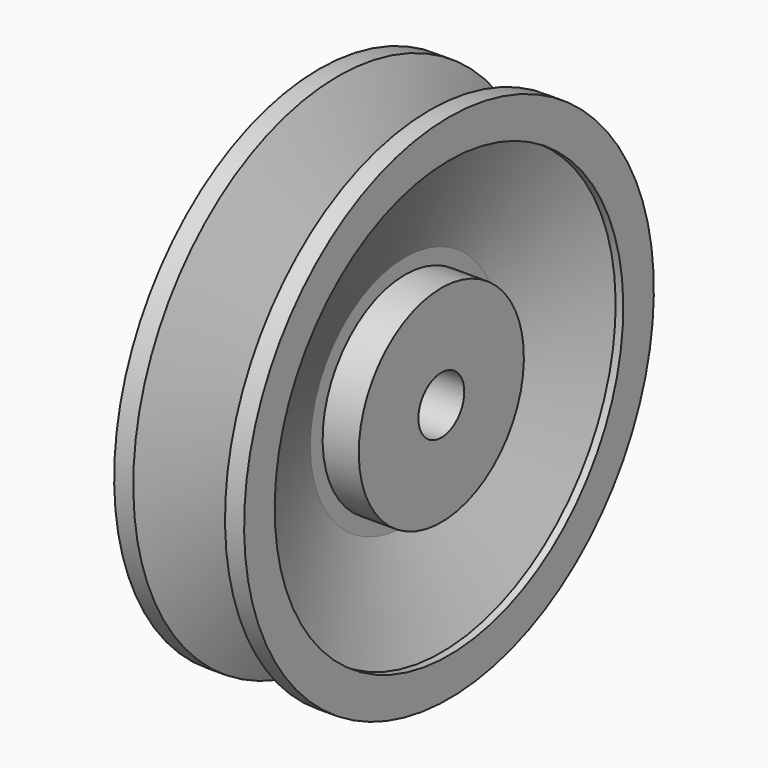
from build123d import *


# Not quite as in the source:
# - a feature names something its author has since deleted; it is built from what else it names


with BuildPart() as f1:
    # F0 (on Front) → F1 (revolve)
    with BuildSketch(Plane.XZ):
        Polygon((-15, 7.5), (0, 7.5), (15, 7.5), (15, 27), (5.5367739091, 27), (5.5367739091, 31), (15, 57), (17, 57), (17, 67), (12, 67), (2.9007441433, 42), (0, 42), (-2.9007441433, 42), (-12, 67), (-17, 67), (-17, 57), (-15, 57), (-5.5367739091, 31), (-5.5367739091, 27), (-15, 27), align=None)
    revolve(axis=Axis((1.6064876985, 0, 0), (1, 0, 0)))


solid = f1.part
